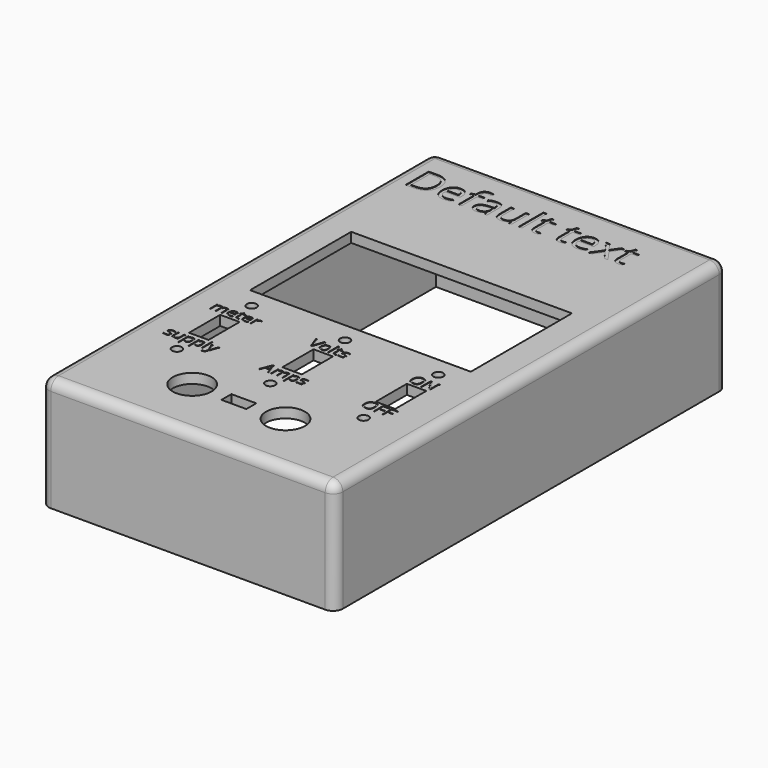
from build123d import *

# Parameters (mm, degrees)
F2_W           = 60
F2_H           = 100
F2_W_2         = 56.2
F2_H_2         = 95.8
F3_DEPTH       = 23
F4_DEPTH       = 21
F5_R           = 2
F1_W           = 45.0453125
F1_H           = 25.796875
F1_W_2         = 3.96875
F1_H_2         = 7.9375
F1_R           = 1
F1_R_2         = 3.96875
F1_W_3         = 5.08
F1_H_3         = 2.54
F6_DEPTH       = 23.001
F7_TEXT_SIZE   = 8.291259615
F7_TEXT_SIZE_2 = 3.4002671096
F8_DEPTH       = 0.1


# Not quite as in the source:
# - Text() gives the source's letters only with a copy of the font that has no kerning and outlines rounded to 1/6400 em; it was checked with that copy


with BuildPart() as f3:
    # F2 (on Top) → F3 (new body)
    with BuildSketch(Plane.XY):
        Rectangle(F2_W, F2_H)
        with Locations((0.3, 0.1)):
            Rectangle(F2_W_2, F2_H_2, mode=Mode.SUBTRACT)
        with Locations((0.3, 0.1)):
            Rectangle(F2_W_2, F2_H_2)
    extrude(amount=F3_DEPTH)

    # F2 (on Top) → F4 (cut)
    with BuildSketch(Plane.XY):
        with Locations((0.3, 0.1)):
            Rectangle(F2_W_2, F2_H_2)
    extrude(amount=F4_DEPTH, mode=Mode.SUBTRACT)

    # F5
    f5_edges = [f3.edges().sort_by_distance(p)[0] for p in [
        (0, -50, 23),
        (30, 0, 23),
        (-30, 0, 23),
        (0, 50, 23),
        (-30, 50, 11.5),
        (-30, -50, 11.5),
        (30, -50, 11.5),
        (30, 50, 11.5),
    ]]
    fillet(f5_edges, radius=F5_R)

    # F1 (on Top) → F6 (cut, through all)
    with BuildSketch(Plane.XY):
        with Locations((-0.09921875, 7.0140625)):
            Rectangle(F1_W, F1_H)
        with Locations((0, -19.471875)):
            Rectangle(F1_W_2, F1_H_2)
        with Locations((0, -9.946875)):
            Circle(F1_R)
        with Locations((0, -28.996875)):
            Circle(F1_R)
        with Locations((-9.525, -37.028125)):
            Circle(F1_R_2)
        with Locations((9.525, -37.028125)):
            Circle(F1_R_2)
        with Locations((0, -37.028125)):
            Rectangle(F1_W_3, F1_H_3)
        with Locations((-19.05, -19.471875)):
            Rectangle(F1_W_2, F1_H_2)
        with Locations((-19.05, -28.996875)):
            Circle(F1_R)
        with Locations((-19.05, -9.946875)):
            Circle(F1_R)
        with Locations((19.05, -9.946875)):
            Circle(F1_R)
        with Locations((19.05, -19.471875)):
            Rectangle(F1_W_2, F1_H_2)
        with Locations((19.05, -28.996875)):
            Circle(F1_R)
    extrude(amount=F6_DEPTH, mode=Mode.SUBTRACT)

    # F7 (on face) → F8 (cut)
    with BuildSketch(Plane.XY.offset(23)):
        with Locations((-26.7783794552, 37.9359610379)):
            Text('Default text', F7_TEXT_SIZE, font='Open Sans', text_align=(TextAlign.LEFT, TextAlign.BOTTOM))
        with Locations((-23.9195544051, -14.8879686099)):
            Text('meter', F7_TEXT_SIZE_2, font='Open Sans', text_align=(TextAlign.LEFT, TextAlign.BOTTOM))
        with Locations((-24.3836377364, -26.2517162337)):
            Text('supply', F7_TEXT_SIZE_2, font='Open Sans', text_align=(TextAlign.LEFT, TextAlign.BOTTOM))
        with Locations((-4.5422786958, -26.2517162337)):
            Text('Amps', F7_TEXT_SIZE_2, font='Open Sans', text_align=(TextAlign.LEFT, TextAlign.BOTTOM))
        with Locations((-3.9121666971, -14.8879686099)):
            Text('Volts', F7_TEXT_SIZE_2, font='Open Sans', text_align=(TextAlign.LEFT, TextAlign.BOTTOM))
        with Locations((16.5008622513, -14.8879686099)):
            Text('ON', F7_TEXT_SIZE_2, font='Open Sans', text_align=(TextAlign.LEFT, TextAlign.BOTTOM))
        with Locations((15.8949240265, -26.2517162337)):
            Text('OFF', F7_TEXT_SIZE_2, font='Open Sans', text_align=(TextAlign.LEFT, TextAlign.BOTTOM))
    extrude(amount=-F8_DEPTH, mode=Mode.SUBTRACT)


solid = f3.part
